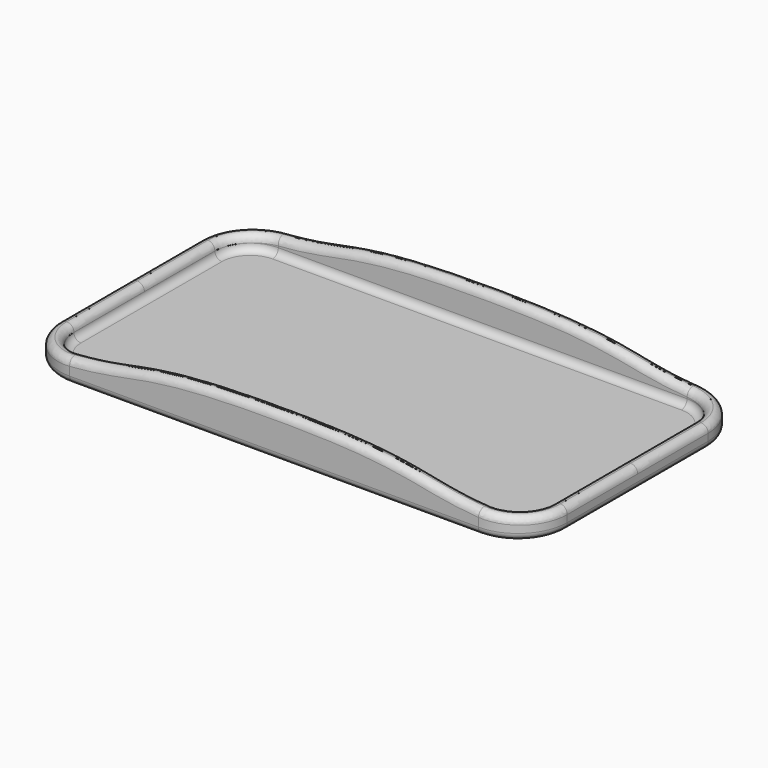
from build123d import *

# Parameters (mm, degrees)
F1_DEPTH = 2
F2_DEPTH = 12
F4_DEPTH = 49.5
F5_R     = 1.9999


# Not quite as in the source:
# - a fillet or chamfer is up to 0.001 mm smaller than in the source, because OpenCascade refuses the exact size


with BuildPart() as f1:
    # F0 (on Top) → F1 (new body)
    with BuildSketch(Plane.XY):
        with BuildLine():
            Line((-58, -35), (58, -35))
            ThreePointArc((58, -35), (65.0710678119, -32.0710678119), (68, -25))
            Line((68, -25), (68, 25))
            ThreePointArc((68, 25), (65.0710678119, 32.0710678119), (58, 35))
            Line((58, 35), (-58, 35))
            ThreePointArc((-58, 35), (-65.0710678119, 32.0710678119), (-68, 25))
            Line((-68, 25), (-68, -25))
            ThreePointArc((-68, -25), (-65.0710678119, -32.0710678119), (-58, -35))
        make_face()
    extrude(amount=F1_DEPTH)

    # F0 (on Top) → F2 (join)
    with BuildSketch(Plane.XY):
        with BuildLine():
            Line((72, -25), (72, 25))
            ThreePointArc((72, 25), (67.8994949366, 34.8994949366), (58, 39))
            Line((58, 39), (-58, 39))
            ThreePointArc((-58, 39), (-67.8994949366, 34.8994949366), (-72, 25))
            Line((-72, 25), (-72, -25))
            ThreePointArc((-72, -25), (-67.8994949366, -34.8994949366), (-58, -39))
            Line((-58, -39), (58, -39))
            ThreePointArc((58, -39), (67.8994949366, -34.8994949366), (72, -25))
        make_face()
        with BuildLine():
            ThreePointArc((68, -25), (65.0710678119, -32.0710678119), (58, -35))
            Line((58, -35), (-58, -35))
            ThreePointArc((-58, -35), (-65.0710678119, -32.0710678119), (-68, -25))
            Line((-68, -25), (-68, 25))
            ThreePointArc((-68, 25), (-65.0710678119, 32.0710678119), (-58, 35))
            Line((-58, 35), (58, 35))
            ThreePointArc((58, 35), (65.0710678119, 32.0710678119), (68, 25))
            Line((68, 25), (68, -25))
        make_face(mode=Mode.SUBTRACT)
    extrude(amount=F2_DEPTH)

    # F3 (on Front) → F4 (intersect, symmetric)
    with BuildSketch(Plane.XZ):
        with BuildLine():
            Line((-72, 0), (72, 0))
            Line((72, 0), (72, 6))
            add(Edge.make_bspline(
                [(72, 6), (37.8172956407, 6), (47.1529476345, 12), (0, 12)],
                knots=[0, 0, 0, 0, 72.2495674728, 72.2495674728, 72.2495674728, 72.2495674728], degree=3))
            add(Edge.make_bspline(
                [(-72, 6), (-37.8172956407, 6), (-47.1529476345, 12), (0, 12)],
                knots=[0, 0, 0, 0, 72.2495674728, 72.2495674728, 72.2495674728, 72.2495674728], degree=3))
            Line((-72, 6), (-72, 0))
        make_face()
    extrude(amount=F4_DEPTH, both=True, mode=Mode.INTERSECT)

    # F5 (radius 2 in the source; OpenCascade refuses exactly that, so slightly less here)
    f5_edges = [f1.edges().sort_by_distance(p)[0] for p in [
        (58, -35, 4.224911),
        (65.071068, -32.071068, 2),
        (68, -25, 4.014778),
        (65.06801, -32.074124, 6.094224),
        (-68, -25, 4.014778),
        (-65.071068, -32.071068, 2),
        (-58, -35, 4.224911),
        (-65.06801, -32.074124, 6.094224),
        (67.899495, 34.899495, 0),
        (58, 39, 3.224911),
        (67.896035, 34.902954, 6.031176),
        (72, 25, 3),
    ]]
    fillet(f5_edges, radius=F5_R)


solid = f1.part
